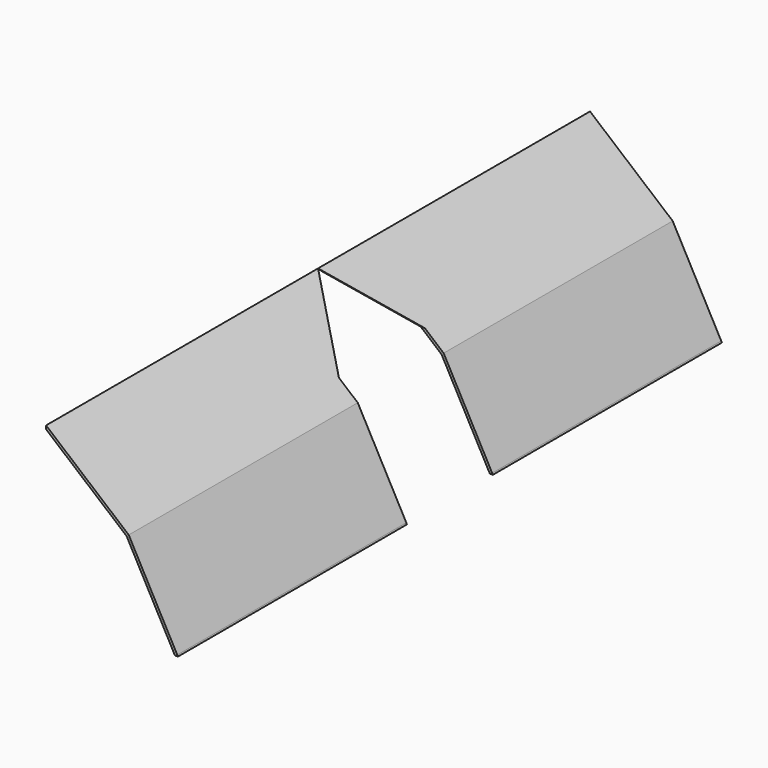
from build123d import *

# Parameters (mm, degrees)
F1_DEPTH  = 247.3
F3_DEPTH  = 300
F4_DEPTH  = 61.9
F5_DEPTH  = 40
F7_DEPTH  = 300
F8_DEPTH  = 300
F10_DEPTH = 300
F11_DEPTH = 25
F12_DEPTH = 71.4
F13_DEPTH = 3
F14_DEPTH = 65.7
F15_DEPTH = 82.2
F2_W      = 20
F2_H      = 39.8570230463
F16_DEPTH = 52.6
F17_DEPTH = 121.6
F18_DEPTH = 3
F20_DEPTH = 25


# Not quite as in the source:
# - a feature of the source that left no trace in its solid (it failed there, or was rolled back) is left out
# - a feature names something its author has since deleted; it is built from what else it names


with BuildPart() as f1:
    # F0 (on Front) → F1 (new body)
    with BuildSketch(Plane.XZ):
        Polygon((-78.8866152354, 43.4383174348), (-78.6296018241, 42.9628188217), (-78.6296018241, 102.819841868), (-127.7663317061, 102.819841868), (-96.9769939736, 76.9071934711), align=None)
        Polygon((-79.7663317061, 42.9628188217), (-97.7663317061, 76.264485822), (-127.7663317061, 101.5128188217), (-157.7663317061, 76.264485822), (-175.7663317061, 42.9628188217), align=None)
        Polygon((-127.7663317061, 101.5128188217), (-97.7663317061, 76.264485822), (-79.7663317061, 42.9628188217), (-78.6296018241, 42.9628188217), (-78.8866152354, 43.4383174348), (-96.9769939736, 76.9071934711), (-127.7663317061, 102.819841868), (-158.5556694386, 76.9071934711), (-176.9030615881, 42.9628188217), (-175.7663317061, 42.9628188217), (-157.7663317061, 76.264485822), align=None)
        Polygon((-176.9030615881, 102.819841868), (-176.9030615881, 42.9628188217), (-158.5556694386, 76.9071934711), (-127.7663317061, 102.819841868), align=None)
    extrude(amount=-F1_DEPTH)

    # F0 (on Front) → F3 (cut)
    with BuildSketch(Plane.XZ):
        Polygon((-78.8866152354, 43.4383174348), (-78.6296018241, 42.9628188217), (-78.6296018241, 102.819841868), (-127.7663317061, 102.819841868), (-96.9769939736, 76.9071934711), align=None)
    extrude(amount=-F3_DEPTH, mode=Mode.SUBTRACT)

    # F2 (on face) → F4 (join)
    with BuildSketch(Plane.YZ.offset(-78.6296018241)):
        Polygon((123.65, 84.6090763807), (123.65, 102.819841868), (103.65, 82.819841868), (123.65, 82.819841868), align=None)
    extrude(amount=-F4_DEPTH)

    # F5 (add): a face of the model
    f5_faces = [f1.faces().sort_by_distance(p)[0] for p in [
        (-91.3159942007, 113.65, 82.819841868),
    ]]
    extrude(f5_faces, amount=F5_DEPTH)

    # F0 (on Front) → F7 (cut)
    with BuildSketch(Plane.XZ):
        Polygon((-79.7663317061, 42.9628188217), (-97.7663317061, 76.264485822), (-127.7663317061, 101.5128188217), (-157.7663317061, 76.264485822), (-175.7663317061, 42.9628188217), align=None)
    extrude(amount=-F7_DEPTH, mode=Mode.SUBTRACT)

    # F0 (on Front) → F8 (cut)
    with BuildSketch(Plane.XZ):
        Polygon((-176.9030615881, 102.819841868), (-176.9030615881, 42.9628188217), (-158.5556694386, 76.9071934711), (-127.7663317061, 102.819841868), align=None)
    extrude(amount=-F8_DEPTH, mode=Mode.SUBTRACT)

    # F9 (on face) → F10 (cut)
    with BuildSketch(Plane.XZ):
        Polygon((-127.7663317061, 101.5128188217), (-127.7663317061, 102.819841868), (-158.5556694386, 76.9071934711), (-176.9030615881, 42.9628188217), (-175.7663317061, 42.9628188217), (-157.7663317061, 76.264485822), align=None)
    extrude(amount=-F10_DEPTH, mode=Mode.SUBTRACT)

    # F11 (cut): a face of the model
    f11_faces = [f1.faces().sort_by_distance(p)[0] for p in [
        (-78.6296018241, 114.3166666667, 68.1531752014),
    ]]
    extrude(f11_faces, amount=-F11_DEPTH, mode=Mode.SUBTRACT)

    # F12 (cut): faces of the model
    f12_faces = [f1.faces().sort_by_distance(p)[0] for p in [
        (-103.6296018241, 116.5184290192, 88.4436749614),
        (-103.6296018241, 113.65, 42.8913303449),
    ]]
    extrude(f12_faces, amount=-F12_DEPTH, mode=Mode.SUBTRACT)

    # F0 (on Front) → F13 (join)
    with BuildSketch(Plane.XZ):
        Polygon((-127.7663317061, 101.5128188217), (-97.7663317061, 76.264485822), (-79.7663317061, 42.9628188217), (-78.6296018241, 42.9628188217), (-78.8866152354, 43.4383174348), (-96.9769939736, 76.9071934711), (-127.7663317061, 102.819841868), (-158.5556694386, 76.9071934711), (-176.9030615881, 42.9628188217), (-175.7663317061, 42.9628188217), (-157.7663317061, 76.264485822), align=None)
    extrude(amount=F13_DEPTH)

    # F2 (on face) → F14 (join)
    with BuildSketch(Plane.YZ.offset(-78.6296018241)):
        Polygon((143.65, 82.819841868), (123.65, 102.819841868), (123.65, 84.6090763807), (123.65, 82.819841868), align=None)
    extrude(amount=-F14_DEPTH)

    # F2 (on face) → F15 (cut)
    with BuildSketch(Plane.YZ.offset(-78.6296018241)):
        Polygon((143.65, 82.819841868), (123.65, 102.819841868), (123.65, 84.6090763807), (123.65, 82.819841868), align=None)
    extrude(amount=-F15_DEPTH, mode=Mode.SUBTRACT)

    # F2 (on face) → F16 (join)
    with BuildSketch(Plane.YZ.offset(-78.6296018241)):
        with Locations((133.65, 62.8913303449)):
            Rectangle(F2_W, F2_H)
    extrude(amount=-F16_DEPTH)

    # F2 (on face) → F17 (cut)
    with BuildSketch(Plane.YZ.offset(-78.6296018241)):
        with Locations((133.65, 62.8913303449)):
            Rectangle(F2_W, F2_H)
    extrude(amount=-F17_DEPTH, mode=Mode.SUBTRACT)

    # F18 (add): a face of the model
    f18_faces = [f1.faces().sort_by_distance(p)[0] for p in [
        (-112.8703238632, 247.3, 89.2710100097),
    ]]
    extrude(f18_faces, amount=F18_DEPTH)

    # F19 (on face) → F20 (cut)
    with BuildSketch(Plane.XZ.offset(3)):
        Polygon((-127.7663317061, 101.5128188217), (-127.7663317061, 102.819841868), (-158.5556694386, 76.9071934711), (-176.9030615881, 42.9628188217), (-175.7663317061, 42.9628188217), (-157.7663317061, 76.264485822), align=None)
    extrude(amount=-F20_DEPTH, mode=Mode.SUBTRACT)


solid = f1.part
